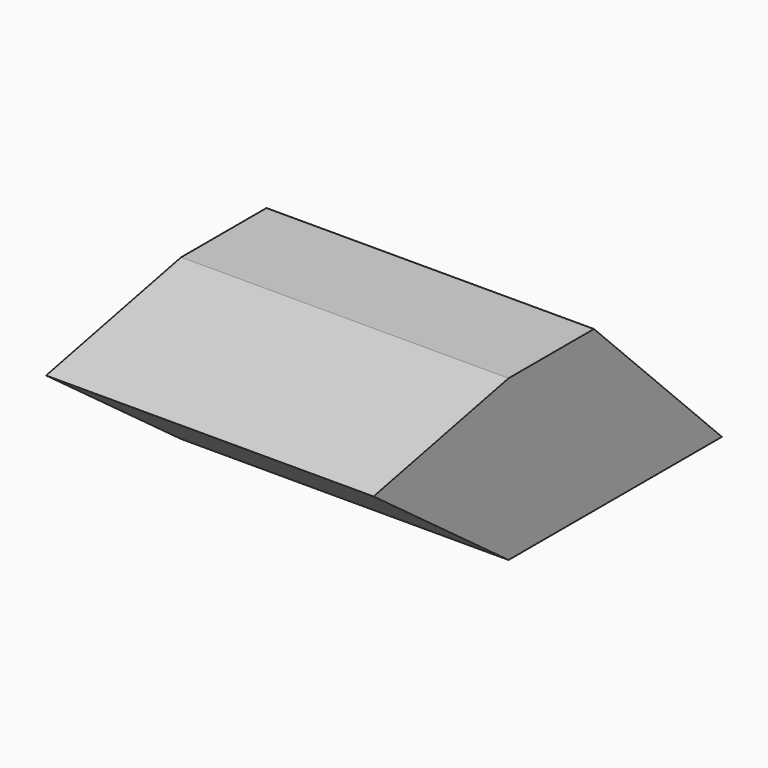
from build123d import *

# Parameters (mm, degrees)
F0_W     = 12.7
F0_H     = 7.62
F1_DEPTH = 15.5956
F2_SIZE  = 7.61999


# Not quite as in the source:
# - a fillet or chamfer is up to 0.001 mm smaller than in the source, because OpenCascade refuses the exact size


with BuildPart() as f1:
    # F0 (on Right) → F1 (new body)
    with BuildSketch(Plane.YZ):
        with Locations((-6.35, 3.81)):
            Rectangle(F0_W, F0_H)
        Polygon((-20.7394696772, 5.931511987), (-12.7, 0), (-12.7, 7.62), align=None)
    extrude(amount=F1_DEPTH)

    # F2 (size 7.62 in the source; OpenCascade refuses exactly that, so slightly less here)
    f2_edges = [f1.edges().sort_by_distance(p)[0] for p in [
        (7.7978, 0, 7.62),
    ]]
    chamfer(f2_edges, length=F2_SIZE)


solid = f1.part
